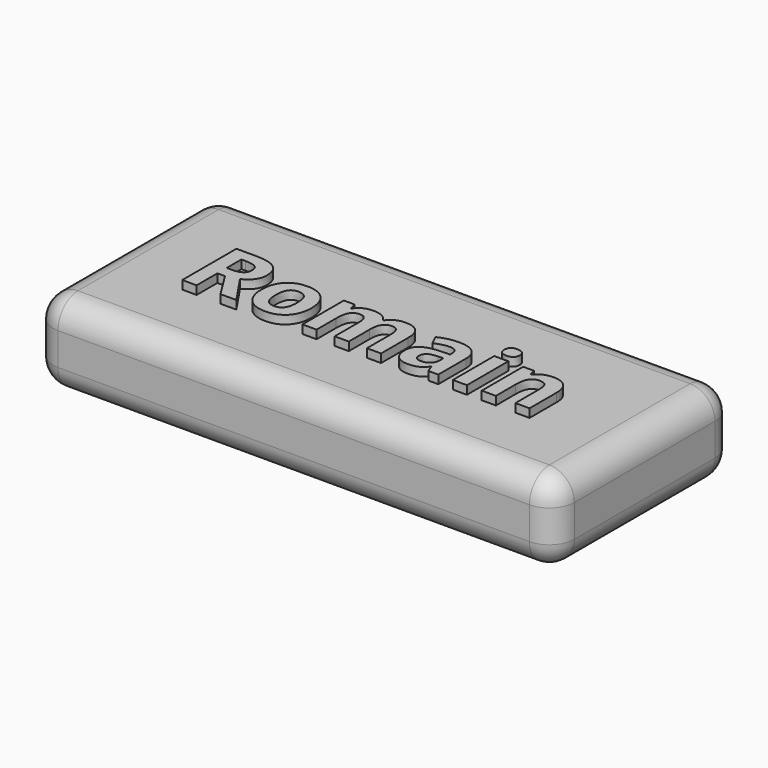
from build123d import *

# Parameters (mm, degrees)
F2_DEPTH     = 16.5
F1_TEXT_SIZE = 19.0034728601
F3_DEPTH     = 18.2
F4_R         = 5


# Not quite as in the source:
# - Text() gives the source's letters only with a copy of the font that has no kerning and outlines rounded to 1/6400 em; it was checked with that copy


with BuildPart() as f2:
    # F0 (on Top) → F2 (new body)
    with BuildSketch(Plane.XY):
        with BuildLine():
            ThreePointArc((52.665643394, 8.9086581767), (51.2011772999, 12.4441920826), (47.665643394, 13.9086581767))
            Line((47.665643394, 13.9086581767), (-46.8189072609, 13.9086581767))
            ThreePointArc((-46.8189072609, 13.9086581767), (-50.3544411668, 12.4441920826), (-51.8189072609, 8.9086581767))
            Line((-51.8189072609, 8.9086581767), (-51.8189072609, -26.3227474689))
            ThreePointArc((-51.8189072609, -26.3227474689), (-50.3544411668, -29.8582813749), (-46.8189072609, -31.3227474689))
            Line((-46.8189072609, -31.3227474689), (47.665643394, -31.3227474689))
            ThreePointArc((47.665643394, -31.3227474689), (51.2011772999, -29.8582813749), (52.665643394, -26.3227474689))
            Line((52.665643394, -26.3227474689), (52.665643394, 8.9086581767))
        make_face()
    extrude(amount=F2_DEPTH)

    # F1 (on Top) → F3 (join)
    with BuildSketch(Plane.XY):
        with Locations((-36.0199378068, -15.8309928956)):
            Text('Romain', F1_TEXT_SIZE, font='Open Sans', font_style=FontStyle.BOLD, text_align=(TextAlign.LEFT, TextAlign.BOTTOM))
    extrude(amount=F3_DEPTH)

    # F4
    f4_edges = [f2.edges().sort_by_distance(p)[0] for p in [
        (0.423368, -31.322747, 16.5),
        (0.423368, -31.322747, 0),
    ]]
    fillet(f4_edges, radius=F4_R)


solid = f2.part
